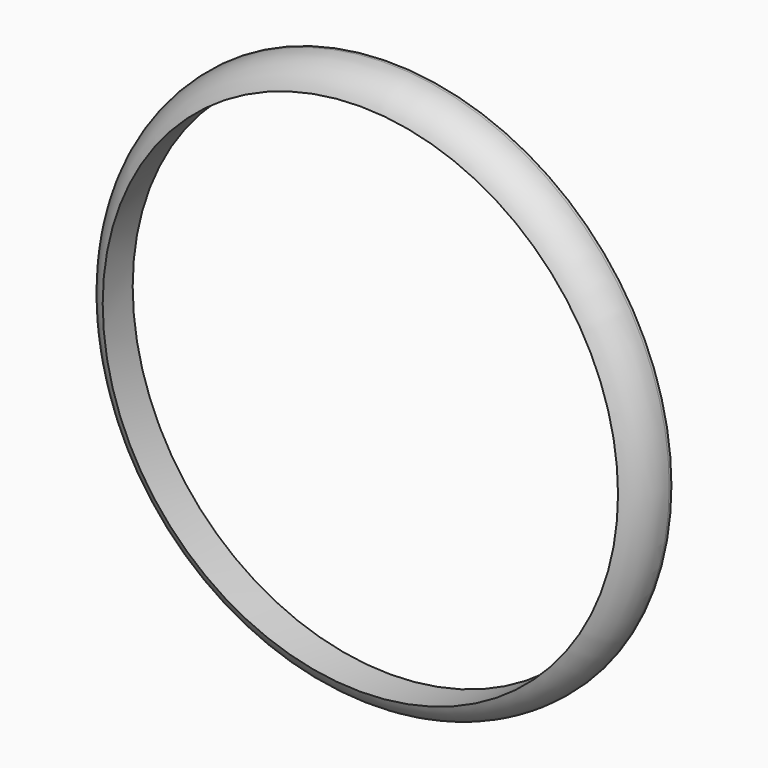
from build123d import *

# Parameters (mm, degrees)
F0_R     = 38.1
F0_R_2   = 34.925
F1_DEPTH = 5.08


# Not quite as in the source:
# - a fillet or chamfer that OpenCascade refuses, or shapes differently, is made with other operations: its cross-section is extruded or revolved along the edge and cut away or added


with BuildPart() as f1:
    # F0 (on Front) → F1 (new body)
    with BuildSketch(Plane.XZ):
        Circle(F0_R)
        Circle(F0_R_2, mode=Mode.SUBTRACT)
    extrude(amount=F1_DEPTH)

    # F2: fillet of radius 5.08 on 1 edges, made by hand

    # F2_s1 → F2_t2 (revolve, cut)
    with BuildSketch(Plane.XY):
        with BuildLine():
            ThreePointArc((38.1, -0.3707139607), (37.2321134838, -3.2105202921), (34.925, -5.08))
            Line((34.925, -5.08), (38.1, -5.08))
            Line((38.1, -5.08), (38.1, -0.3707139607))
        make_face()
    revolve(axis=Axis((0, -5.08, 0), (0, -1, 0)), mode=Mode.SUBTRACT)


solid = f1.part
